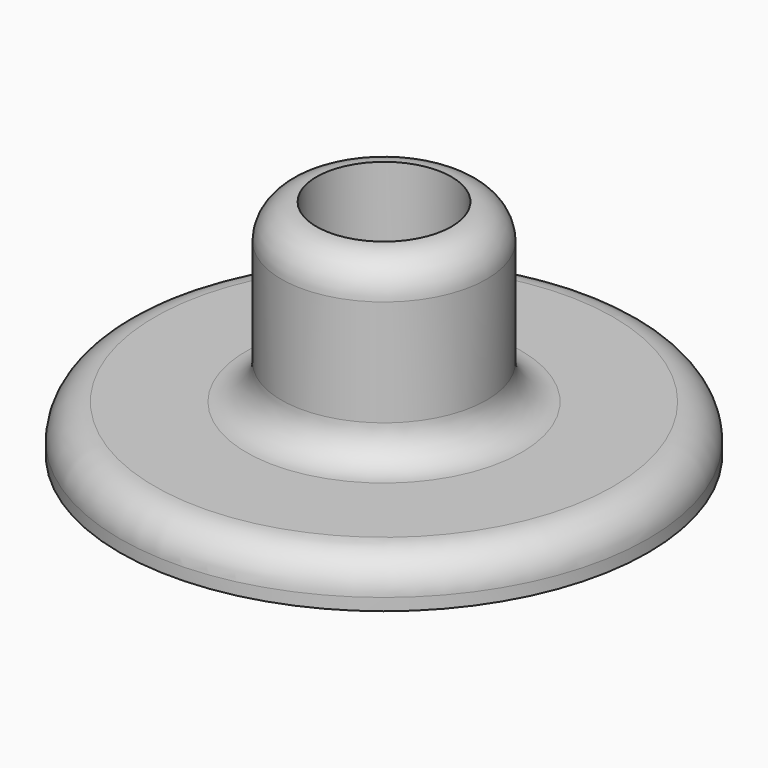
from build123d import *

# Parameters (mm, degrees)
F0_R     = 45
F0_R_2   = 7.075
F1_DEPTH = 8
F2_R     = 17.5
F2_R_2   = 11.5
F3_DEPTH = 30


# Not quite as in the source:
# - a fillet or chamfer that OpenCascade refuses, or shapes differently, is made with other operations: its cross-section is extruded or revolved along the edge and cut away or added


with BuildPart() as f1:
    # F0 (on Top) → F1 (new body)
    with BuildSketch(Plane.XY):
        Circle(F0_R)
        Circle(F0_R_2, mode=Mode.SUBTRACT)
    extrude(amount=F1_DEPTH)

    # F2 (on face) → F3 (join)
    with BuildSketch(Plane.XY.offset(8)):
        Circle(F2_R)
        Circle(F2_R_2, mode=Mode.SUBTRACT)
    extrude(amount=F3_DEPTH)

    # F4: fillet of radius 6 on 4 edges, made by hand

    # F4_s1 → F4_t2 (revolve)
    with BuildSketch(Plane.XZ):
        with BuildLine():
            ThreePointArc((23.5009656854, 7.9996), (19.2573593129, 9.7573593129), (17.4996, 14.0009656854))
            Line((17.4996, 14.0009656854), (16.8994634315, 14.0009656854))
            ThreePointArc((16.8994634315, 14.0009656854), (16.8998634315, 11.0004828427), (16.8998634315, 8))
            Line((16.8998634315, 8), (17.5, 7.3998634315))
            ThreePointArc((17.5, 7.3998634315), (20.5004828427, 7.3998634315), (23.5009656854, 7.3994634315))
            Line((23.5009656854, 7.3994634315), (23.5009656854, 7.9996))
        make_face()
    revolve(axis=Axis((0, 0, 8), (0, 0, 1)))

    # F4_s3 → F4_t4 (revolve)
    with BuildSketch(Plane.XZ):
        with BuildLine():
            ThreePointArc((7.0751050475, 7.9996140401), (10.2674180504, 10.1463065699), (11.5004, 13.7903299833))
            Line((11.5004, 13.7903299833), (12.1005365685, 13.7903299833))
            ThreePointArc((12.1005365685, 13.7903299833), (12.1001365685, 10.8951649917), (12.1001365685, 8))
            Line((12.1001365685, 8), (11.5, 7.3998634315))
            ThreePointArc((11.5, 7.3998634315), (9.2875525237, 7.3998634315), (7.2327121208, 7.4205424458))
            Line((7.2327121208, 7.4205424458), (7.0751050475, 7.9996140401))
        make_face()
    revolve(axis=Axis((0, 0, 8), (0, 0, 1)))

    # F4_s5 → F4_t6 (revolve, cut)
    with BuildSketch(Plane.XZ):
        with BuildLine():
            ThreePointArc((45.0004, 1.9990343146), (43.2426406871, 6.2426406871), (38.9990343146, 8.0004))
            Line((38.9990343146, 8.0004), (38.9990343146, 8.6005365685))
            ThreePointArc((38.9990343146, 8.6005365685), (41.9995171573, 8.6001365685), (45, 8.6001365685))
            Line((45, 8.6001365685), (45.6001365685, 8))
            ThreePointArc((45.6001365685, 8), (45.6001365685, 4.9995171573), (45.6005365685, 1.9990343146))
            Line((45.6005365685, 1.9990343146), (45.0004, 1.9990343146))
        make_face()
    revolve(axis=Axis((0, 0, 8), (0, 0, 1)), mode=Mode.SUBTRACT)

    # F4_s7 → F4_t8 (revolve, cut)
    with BuildSketch(Plane.XZ):
        with BuildLine():
            ThreePointArc((17.5004, 31.9990343923), (15.7429821175, 36.242299307), (11.5000000644, 38.0004))
            Line((11.5000000644, 38.0004), (11.5000966393, 38.6005365608))
            ThreePointArc((11.5000966393, 38.6005365608), (14.5000000322, 38.6001365685), (17.5, 38.6001365685))
            Line((17.5, 38.6001365685), (18.1001365685, 38))
            ThreePointArc((18.1001365685, 38), (18.1001365685, 34.9995171961), (18.1005365685, 31.9990343923))
            Line((18.1005365685, 31.9990343923), (17.5004, 31.9990343923))
        make_face()
    revolve(axis=Axis((0, 0, 38), (0, 0, 1)), mode=Mode.SUBTRACT)


solid = f1.part
